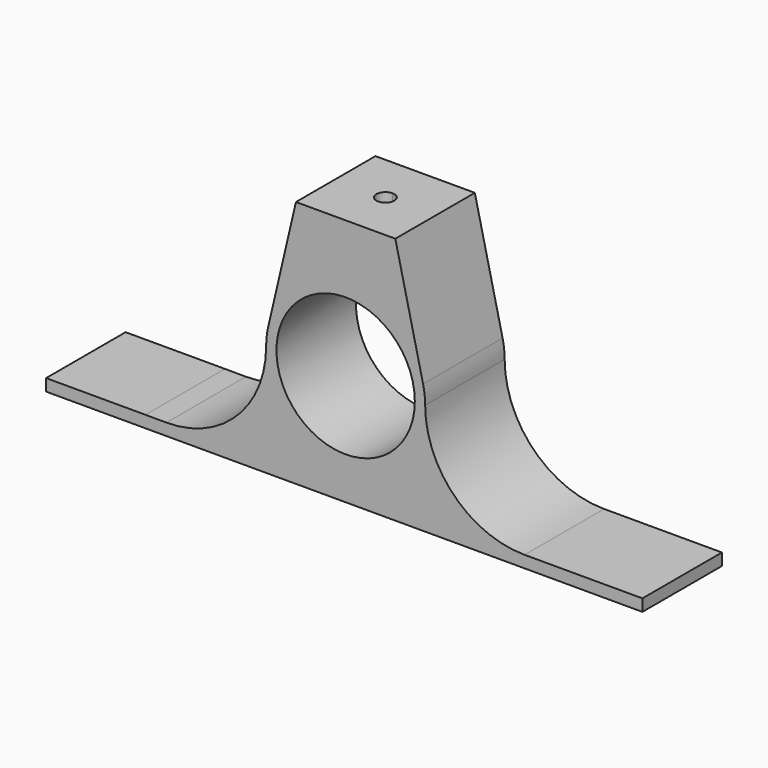
from build123d import *

# Parameters (mm, degrees)
F0_R     = 17.4
F1_DEPTH = 25
F3_DEPTH = 50


# Not quite as in the source:
# - ends of sketch curves that miss each other by under 0.0002 mm in the source are joined


with BuildPart() as f1:
    # F0 (on Front) → F1 (new body)
    with BuildSketch(Plane.XZ):
        with BuildLine():
            ThreePointArc((-19.4763321764, 4.5467004469), (0, 20), (19.4763321764, 4.5467004469))
            Line((19.4763321764, 4.5467004469), (12.5, 34.4306491315))
            Line((12.5, 34.4306491315), (0, 34.4306491315))
            Line((0, 34.4306491315), (-12.5, 34.4306491315))
            Line((-12.5, 34.4306491315), (-19.4763321764, 4.5467004469))
        make_face()
        with BuildLine():
            ThreePointArc((-19.9999883661, -0.0215721294), (0.0107860663, -19.9999970915), (20, 0))
            ThreePointArc((20, 0), (19.8686517349, 2.2883789537), (19.4763321764, 4.5467004469))
            ThreePointArc((19.4763321764, 4.5467004469), (0, 20), (-19.4763321764, 4.5467004469))
            ThreePointArc((-19.4763321764, 4.5467004469), (-19.8686517349, 2.2883789537), (-20, 0))
            ThreePointArc((-20, 0), (-19.9999970915, -0.0107860663), (-19.9999883661, -0.0215721294))
        make_face()
        Circle(F0_R, mode=Mode.SUBTRACT)
        with BuildLine():
            ThreePointArc((45, -25), (27.3223304703, -17.6776695297), (20, 0))
            ThreePointArc((20, 0), (0.0107860663, -19.9999970915), (-19.9999883661, -0.0215721294))
            ThreePointArc((-19.9999883661, -0.0215721294), (-27.3583172251, -17.7351553161), (-45.1016823096, -25.0213653552))
            Line((-45.1016823096, -25.0213653552), (-50.3546064898, -25))
            Line((-50.3546064898, -25), (-75.3500018494, -25))
            Line((-75.3500018494, -25), (-75.3500018494, -28))
            Line((-75.3500018494, -28), (74.6500011308, -28))
            Line((74.6500011308, -28), (74.65, -25))
            Line((74.65, -25), (50.3546064898, -25))
            Line((50.3546064898, -25), (45, -25))
        make_face()
    extrude(amount=F1_DEPTH)

    # F2 (on face) → F3 (cut)
    with BuildSketch(Plane.XY.offset(34.4306491315)):
        with BuildLine():
            ThreePointArc((2.25, -12.5), (1.5909902577, -10.9090097423), (0, -10.25))
            ThreePointArc((0, -10.25), (-1.5909902577, -14.0909902577), (2.25, -12.5))
        make_face()
    extrude(amount=-F3_DEPTH, mode=Mode.SUBTRACT)


solid = f1.part
